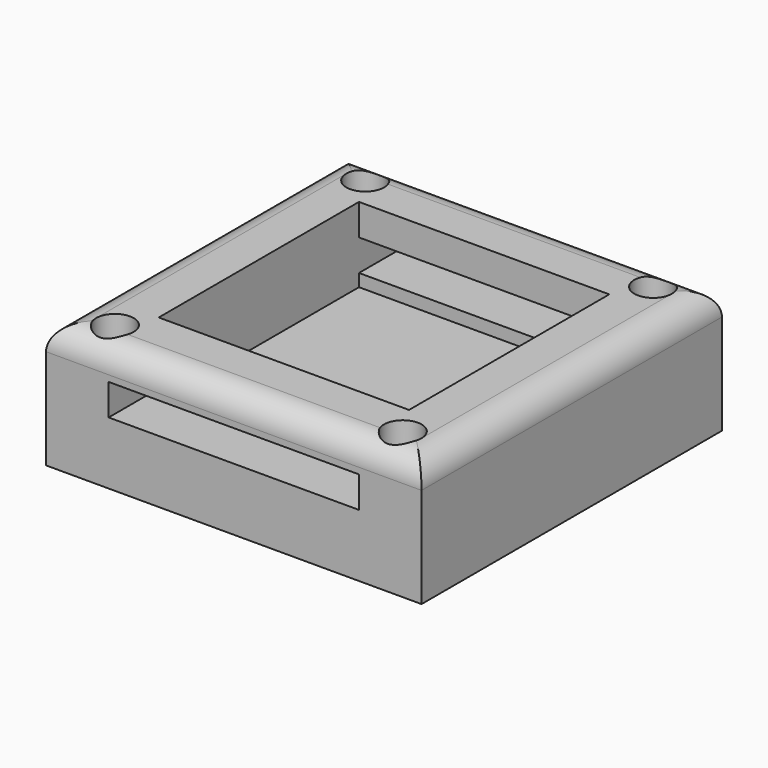
from build123d import *

# Parameters (mm, degrees)
F0_W        = 76.2
F0_H        = 76.2
F1_DEPTH    = 25.4
F2_W        = 50.8
F2_H        = 6.35
F3_DEPTH    = 76.201
F4_W        = 50.8
F4_H        = 50.8
F5_DEPTH    = 15.24
F6_R        = 3.81
F7_DEPTH    = 5.08
F8_T1_DEPTH = 101.6
F8_T3_DEPTH = 101.6


# Not quite as in the source:
# - a fillet or chamfer that OpenCascade refuses, or shapes differently, is made with other operations: its cross-section is extruded or revolved along the edge and cut away or added


with BuildPart() as f1:
    # F0 (on Top) → F1 (new body)
    with BuildSketch(Plane.XY):
        with Locations((9.967116639, 1.2604303423)):
            Rectangle(F0_W, F0_H)
    extrude(amount=F1_DEPTH)

    # F2 (on face) → F3 (cut, through all)
    with BuildSketch(Plane.XZ.offset(36.8395696577)):
        with Locations((9.967116639, 15.875)):
            Rectangle(F2_W, F2_H)
    extrude(amount=-F3_DEPTH, mode=Mode.SUBTRACT)

    # F4 (on face) → F5 (cut)
    with BuildSketch(Plane.XY.offset(25.4)):
        with Locations((9.967116639, 1.2604303423)):
            Rectangle(F4_W, F4_H)
    extrude(amount=-F5_DEPTH, mode=Mode.SUBTRACT)

    # F6 (on face) → F7 (cut)
    with BuildSketch(Plane.XY.offset(25.4)):
        with Locations((-19.242883361, 33.0104303423)):
            Circle(F6_R)
        with Locations((39.177116639, 33.0104303423)):
            Circle(F6_R)
        with Locations((-19.242883361, -30.4895696577)):
            Circle(F6_R)
        with Locations((39.177116639, -30.4895696577)):
            Circle(F6_R)
    extrude(amount=-F7_DEPTH, mode=Mode.SUBTRACT)

    # F8: fillet of radius 5.08 on 4 edges, made by hand

    # F8_s2 → F8_t1 (cut)
    with BuildSketch(Plane.XZ.offset(-52.0604303423)):
        with BuildLine():
            ThreePointArc((48.067116639, 20.32), (46.5792190874, 23.9121024484), (42.987116639, 25.4))
            Line((42.987116639, 25.4), (48.067116639, 25.4))
            Line((48.067116639, 25.4), (48.067116639, 20.32))
        make_face()
        with BuildLine():
            ThreePointArc((-23.052883361, 25.4), (-26.6449858094, 23.9121024484), (-28.132883361, 20.32))
            Line((-28.132883361, 20.32), (-28.132883361, 25.4))
            Line((-28.132883361, 25.4), (-23.052883361, 25.4))
        make_face()
    extrude(amount=F8_T1_DEPTH, mode=Mode.SUBTRACT)

    # F8_s4 → F8_t3 (cut)
    with BuildSketch(Plane.YZ.offset(-40.832883361)):
        with BuildLine():
            ThreePointArc((-31.7595696577, 25.4), (-35.3516721061, 23.9121024484), (-36.8395696577, 20.32))
            Line((-36.8395696577, 20.32), (-36.8395696577, 25.4))
            Line((-36.8395696577, 25.4), (-31.7595696577, 25.4))
        make_face()
        with BuildLine():
            ThreePointArc((39.3604303423, 20.32), (37.8725327907, 23.9121024484), (34.2804303423, 25.4))
            Line((34.2804303423, 25.4), (39.3604303423, 25.4))
            Line((39.3604303423, 25.4), (39.3604303423, 20.32))
        make_face()
    extrude(amount=F8_T3_DEPTH, mode=Mode.SUBTRACT)


solid = f1.part
